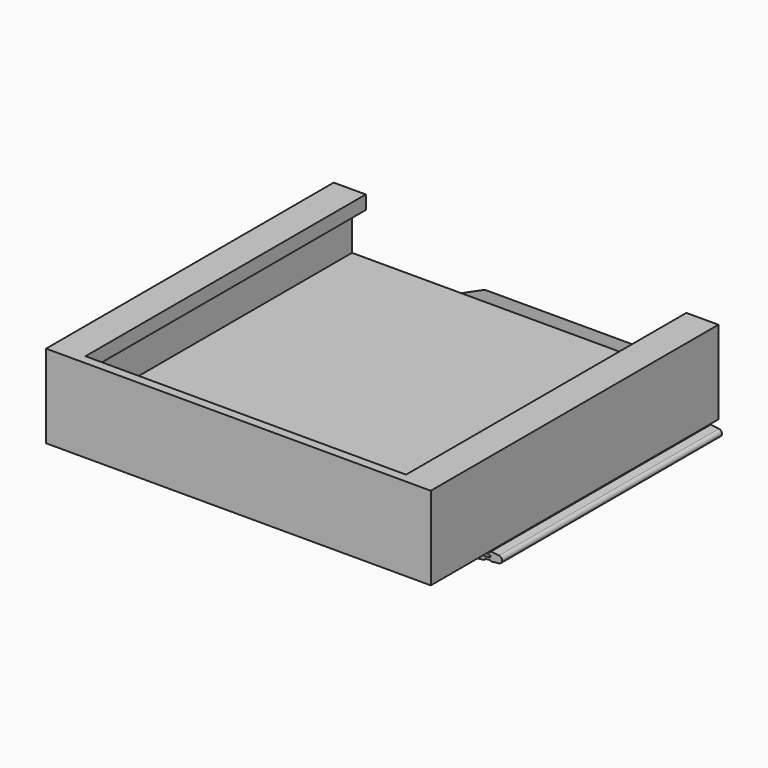
from build123d import *

# Parameters (mm, degrees)
F1_DEPTH      = 76.5
F3_DEPTH      = 60
F4_W          = 84
F4_H          = 2
F5_DEPTH      = 12.2
F5_DEPTH_BACK = 6
F7_DEPTH      = 25
F7_DEPTH_BACK = 25
F8_W          = 50
F8_H          = 8
F9_ANGLE_BACK = 45
F9_ANGLE      = 90
F10_T4_DEPTH  = 68.2385540506
F10_T9_DEPTH  = 68.2385540506
F11_W         = 5
F11_H         = 1.5
F14_DEPTH     = 60
F15_F1_R      = 0.75
F15_F2_R      = 0.75


# Not quite as in the source:
# - a fillet or chamfer that OpenCascade refuses, or shapes differently, is made with other operations: its cross-section is extruded or revolved along the edge and cut away or added


with BuildPart() as f1:
    # F0 (on Front) → F1 (new body)
    with BuildSketch(Plane.XZ):
        Polygon((-35, 9.2), (-35, 12.2), (-42, 12.2), (-42, -6), (0, -6), (42, -6), (42, 12.2), (35, 12.2), (35, 9.2), (38, 9.2), (38, 0), (0, 0), (-38, 0), (-38, 9.2), align=None)
    extrude(amount=F1_DEPTH)

    # F2 (on Front) → F3 (join)
    with BuildSketch(Plane.XZ):
        Polygon((-40, -8.5), (-20, -6), (-28.0622577483, -6), (-48.0622577483, -8.5), (-28.0622577483, -11), (-28.0622577483, -16), (0, -16), (28.0622577483, -16), (28.0622577483, -11), (48.0622577483, -8.5), (28.0622577483, -6), (20, -6), (40, -8.5), (20, -11), (0, -11), (-20, -11), align=None)
    extrude(amount=F3_DEPTH)

    # F4 (on face) → F5 (join, two sides)
    with BuildSketch(Plane.XY) as f5_sk:
        with Locations((0, -77.5)):
            Rectangle(F4_W, F4_H)
    extrude(amount=F5_DEPTH)
    extrude(f5_sk.sketch, amount=-F5_DEPTH_BACK)

    # F6 (on Right) → F7 (join, two sides)
    with BuildSketch(Plane.YZ) as f7_sk:
        Polygon((0, -14.9692235936), (0, -16), (20, -11), (0, -4.9240960793), (0, -5.9692235936), (16.2514952539, -10.9063497801), align=None)
        Polygon((-20, -11), (0, -16), (0, -14.9692235936), (-16.2514952539, -10.9063497801), (0, -5.9692235936), (0, -4.9240960793), align=None)
    extrude(amount=F7_DEPTH)
    extrude(f7_sk.sketch, amount=-F7_DEPTH_BACK)

    # F8 (on Right) → F9 (revolve)
    with BuildSketch(Plane.YZ, mode=Mode.PRIVATE) as f9_sk:
        with Locations((-22, -15)):
            Rectangle(F8_W, F8_H)
    revolve(f9_sk.sketch.rotate(Axis((0, -22, -39), (0, 1, 0)), -F9_ANGLE_BACK), axis=Axis((0, -22, -39), (0, 1, 0)), revolution_arc=F9_ANGLE)

    # F10: fillet of radius 5 on 2 edges, made by hand


with BuildPart() as f10_tool2:
    # F10_s3 → F10_t4 (new body)
    with BuildSketch(Plane.XZ.offset(-21.2385540506)):
        with BuildLine():
            ThreePointArc((-19.7989898732, -19.2010101268), (-21.6352675362, -16.8772006254), (-24.4641410429, -16))
            Line((-24.4641410429, -16), (-15.9687194227, -16))
            ThreePointArc((-15.9687194227, -16), (-17.9553299476, -17.5149790209), (-19.7989898732, -19.2010101268))
        make_face()
    extrude(amount=F10_T4_DEPTH)

    split(bisect_by=Plane(origin=(0, 3.7647058824, -15.0588235294), x_dir=(1, 0, 0), z_dir=(0, -0.242535625, 0.9701425001)), keep=Keep.TOP)


with BuildPart() as f1_1:
    add(f1.part)

    # F10_t1: union F10_tool2
    add(f10_tool2.part)


with BuildPart() as f10_tool7:
    # F10_s8 → F10_t9 (new body)
    with BuildSketch(Plane.XZ.offset(-21.2385540506)):
        with BuildLine():
            ThreePointArc((19.7989898732, -19.2010101268), (21.6352675362, -16.8772006254), (24.4641410429, -16))
            Line((24.4641410429, -16), (15.9687194227, -16))
            ThreePointArc((15.9687194227, -16), (17.9553299476, -17.5149790209), (19.7989898732, -19.2010101268))
        make_face()
    extrude(amount=F10_T9_DEPTH)

    split(bisect_by=Plane(origin=(0, 3.7647058824, -15.0588235294), x_dir=(1, 0, 0), z_dir=(0, -0.242535625, 0.9701425001)), keep=Keep.TOP)


with BuildPart() as f1_2:
    add(f1_1.part)

    # F10_t6: union F10_tool7
    add(f10_tool7.part)

    # F11 (on Right) → F12 (revolve, cut)
    with BuildSketch(Plane.YZ):
        with Locations((-51.5, -15.75)):
            Rectangle(F11_W, F11_H)
        with Locations((-46.5, -15.75)):
            Rectangle(F11_W, F11_H)
    revolve(axis=Axis((0, -22, -34.8578643763), (0, 1, 0)), mode=Mode.SUBTRACT)

    # F13 (on face) → F14 (cut, through all)
    with BuildSketch(Plane.XZ.offset(60)):
        with BuildLine():
            Line((38.9456393414, -8.8837402215), (40, -8.75))
            ThreePointArc((40, -8.75), (40.25, -8.5), (40, -8.25))
            Line((40, -8.25), (39.0077436029, -8.1257935491))
            ThreePointArc((39.0077436029, -8.1257935491), (38.8060744602, -8.1623581433), (38.6995205721, -8.3374400715))
            Line((38.6995205721, -8.3374400715), (38.6661107322, -8.6047187912))
            ThreePointArc((38.6661107322, -8.6047187912), (38.737564097, -8.8126646153), (38.9456393414, -8.8837402215))
        make_face()
        with BuildLine():
            Line((39.0699789435, -7.627910704), (40.0622568202, -7.7519454386))
            ThreePointArc((40.0622568202, -7.7519454386), (40.341334973, -7.5348846531), (40.1242741875, -7.2558065003))
            Line((40.1242741875, -7.2558065003), (39.1319963108, -7.1317717657))
            ThreePointArc((39.1319963108, -7.1317717657), (38.8529181579, -7.3488325512), (39.0699789435, -7.627910704))
        make_face()
        with BuildLine():
            Line((29.054535625, -5.8740347346), (28.0622577483, -5.75))
            ThreePointArc((28.0622577483, -5.75), (27.8141882791, -5.9689913164), (28.0007192868, -6.2423076923))
            Line((28.0007192868, -6.2423076923), (28.9929971635, -6.3663424269))
            ThreePointArc((28.9929971635, -6.3663424269), (29.2699202404, -6.1509578115), (29.054535625, -5.8740347346))
        make_face()
        with BuildLine():
            Line((28.9307403433, -6.8643969883), (27.9384624666, -6.7403622537))
            ThreePointArc((27.9384624666, -6.7403622537), (27.6593843138, -6.9574230392), (27.8764450993, -7.236501192))
            Line((27.8764450993, -7.236501192), (28.868722976, -7.3605359266))
            ThreePointArc((28.868722976, -7.3605359266), (29.1478011288, -7.1434751411), (28.9307403433, -6.8643969883))
        make_face()
        with BuildLine():
            ThreePointArc((39.0699789435, -9.372089296), (38.8529181579, -9.6511674488), (39.1319963108, -9.8682282343))
            Line((39.1319963108, -9.8682282343), (40.1242741875, -9.7441934997))
            ThreePointArc((40.1242741875, -9.7441934997), (40.341334973, -9.4651153469), (40.0622568202, -9.2480545614))
            Line((40.0622568202, -9.2480545614), (39.0699789435, -9.372089296))
        make_face()
        with BuildLine():
            Line((27.9384624666, -10.2596377463), (28.9307403433, -10.1356030117))
            ThreePointArc((28.9307403433, -10.1356030117), (29.1478011288, -9.8565248589), (28.868722976, -9.6394640734))
            Line((28.868722976, -9.6394640734), (27.8764450993, -9.763498808))
            ThreePointArc((27.8764450993, -9.763498808), (27.6593843138, -10.0425769608), (27.9384624666, -10.2596377463))
        make_face()
        with BuildLine():
            ThreePointArc((28.0007192868, -10.7576923077), (27.8141882791, -11.0310086836), (28.0622577483, -11.25))
            Line((28.0622577483, -11.25), (29.054535625, -11.1259652654))
            ThreePointArc((29.054535625, -11.1259652654), (29.2699202404, -10.8490421885), (28.9929971635, -10.6336575731))
            Line((28.9929971635, -10.6336575731), (28.0007192868, -10.7576923077))
        make_face()
        with BuildLine():
            Line((-38.6661107322, -8.6047187912), (-38.6995205721, -8.3374400715))
            ThreePointArc((-38.6995205721, -8.3374400715), (-38.8060744602, -8.1623581433), (-39.0077436029, -8.1257935491))
            Line((-39.0077436029, -8.1257935491), (-40, -8.25))
            ThreePointArc((-40, -8.25), (-40.25, -8.5), (-40, -8.75))
            Line((-40, -8.75), (-38.9456393414, -8.8837402215))
            ThreePointArc((-38.9456393414, -8.8837402215), (-38.737564097, -8.8126646153), (-38.6661107322, -8.6047187912))
        make_face()
        with BuildLine():
            Line((-40.0622568202, -7.7519454386), (-39.0699789435, -7.627910704))
            ThreePointArc((-39.0699789435, -7.627910704), (-38.8529181579, -7.3488325512), (-39.1319963108, -7.1317717657))
            Line((-39.1319963108, -7.1317717657), (-40.1242741875, -7.2558065003))
            ThreePointArc((-40.1242741875, -7.2558065003), (-40.341334973, -7.5348846531), (-40.0622568202, -7.7519454386))
        make_face()
        with BuildLine():
            ThreePointArc((-39.1319963108, -9.8682282343), (-38.8529181579, -9.6511674488), (-39.0699789435, -9.372089296))
            Line((-39.0699789435, -9.372089296), (-40.0622568202, -9.2480545614))
            ThreePointArc((-40.0622568202, -9.2480545614), (-40.341334973, -9.4651153469), (-40.1242741875, -9.7441934997))
            Line((-40.1242741875, -9.7441934997), (-39.1319963108, -9.8682282343))
        make_face()
        with BuildLine():
            ThreePointArc((-28.0007192868, -6.2423076923), (-27.8141882791, -5.9689913164), (-28.0622577483, -5.75))
            Line((-28.0622577483, -5.75), (-29.054535625, -5.8740347346))
            ThreePointArc((-29.054535625, -5.8740347346), (-29.2699202404, -6.1509578115), (-28.9929971635, -6.3663424269))
            Line((-28.9929971635, -6.3663424269), (-28.0007192868, -6.2423076923))
        make_face()
        with BuildLine():
            ThreePointArc((-27.9384624666, -10.2596377463), (-27.6593843138, -10.0425769608), (-27.8764450993, -9.763498808))
            Line((-27.8764450993, -9.763498808), (-28.868722976, -9.6394640734))
            ThreePointArc((-28.868722976, -9.6394640734), (-29.1478011288, -9.8565248589), (-28.9307403433, -10.1356030117))
            Line((-28.9307403433, -10.1356030117), (-27.9384624666, -10.2596377463))
        make_face()
        with BuildLine():
            ThreePointArc((-28.0622577483, -11.25), (-27.8141882791, -11.0310086836), (-28.0007192868, -10.7576923077))
            Line((-28.0007192868, -10.7576923077), (-28.9929971635, -10.6336575731))
            ThreePointArc((-28.9929971635, -10.6336575731), (-29.2699202404, -10.8490421885), (-29.054535625, -11.1259652654))
            Line((-29.054535625, -11.1259652654), (-28.0622577483, -11.25))
        make_face()
        with BuildLine():
            ThreePointArc((-27.8764450993, -7.236501192), (-27.6593843138, -6.9574230392), (-27.9384624666, -6.7403622537))
            Line((-27.9384624666, -6.7403622537), (-28.9307403433, -6.8643969883))
            ThreePointArc((-28.9307403433, -6.8643969883), (-29.1478011288, -7.1434751411), (-28.868722976, -7.3605359266))
            Line((-28.868722976, -7.3605359266), (-27.8764450993, -7.236501192))
        make_face()
    extrude(amount=-F14_DEPTH, mode=Mode.SUBTRACT)

    # F15: fillet of radius 0.75 on 2 edges, made by hand

    # F15_f1
    f15_f1_edges = [f1_2.edges().sort_by_distance(p)[0] for p in [
        (-48.0622577483, -30, -8.5),
    ]]
    fillet(f15_f1_edges, radius=F15_F1_R)

    # F15_f2
    f15_f2_edges = [f1_2.edges().sort_by_distance(p)[0] for p in [
        (48.0622577483, -30, -8.5),
    ]]
    fillet(f15_f2_edges, radius=F15_F2_R)


solid = f1_2.part
